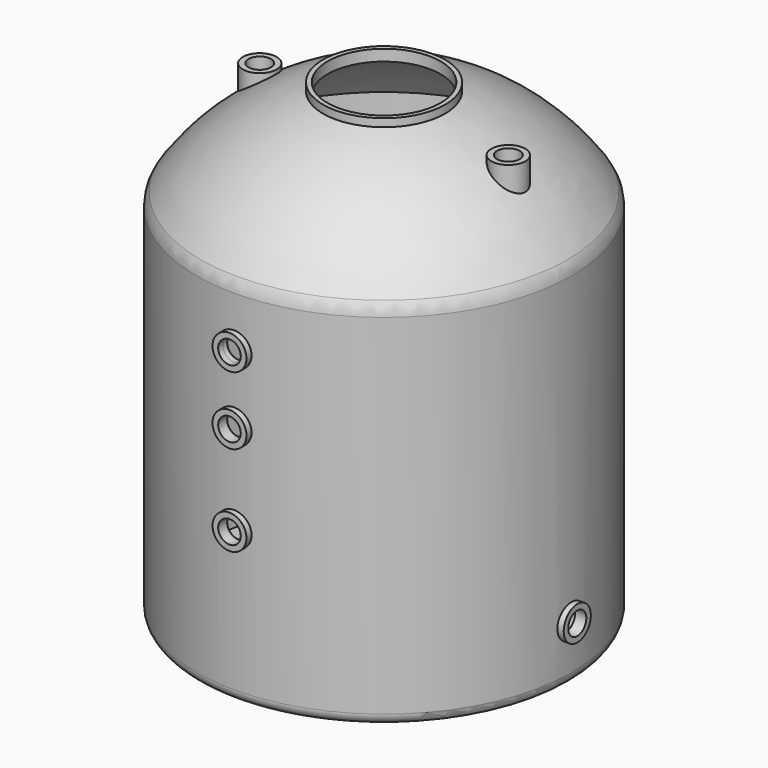
from build123d import *

# Parameters (mm, degrees)
F3_T      = 2
F9_DEPTH  = 12.5
F12_R     = 5
F13_DEPTH = 12.5
F14_R     = 7.5
F14_R_2   = 5
F15_DEPTH = 2.5
F19_R     = 10
F20_R     = 5
F24_R     = 5
F25_DEPTH = 40
F28_R     = 7.5
F28_R_2   = 5
F29_DEPTH = 10
F18_R     = 5
F30_DEPTH = 2.1554683744
F31_R     = 7.5
F31_R_2   = 5
F32_DEPTH = 2.5
F33_R     = 5
F34_DEPTH = 2.1554683744
F35_R     = 7.5
F35_R_2   = 5
F36_DEPTH = 2.5
F38_R     = 5
F39_DEPTH = 2.1554683744
F40_R     = 7.5
F40_R_2   = 5
F41_DEPTH = 2.5
F42_W     = 2.5
F42_H     = 1.25
F43_DEPTH = 3


with BuildPart() as f1:
    # F0 (on Front) → F1 (revolve)
    with BuildSketch(Plane.XZ):
        with BuildLine():
            Line((25, 99.9657286556), (0, 99.9657286556))
            Line((0, 99.9657286556), (0, -106.0342713444))
            Line((0, -106.0342713444), (81, -106.0342713444))
            Line((81, -106.0342713444), (81, 53.9657286556))
            ThreePointArc((81, 53.9657286556), (56.6710521362, 79.4798486465), (25, 94.9657286556))
            Line((25, 94.9657286556), (25, 99.9657286556))
        make_face()
    revolve(axis=Axis((0, 0, -3.0342713444), (0, 0, -1)))

    # F3
    f3_openings = [f1.faces().sort_by_distance(p)[0] for p in [
        (0, 0, 99.965729),
    ]]
    offset(amount=F3_T, openings=f3_openings, kind=Kind.INTERSECTION)

    # F8 (on offset) → F9 (cut, symmetric)
    with BuildSketch(Plane.XY.offset(61.5641335174)):
        with BuildLine():
            ThreePointArc((-43.2126436782, -4.9917358047), (-39.8642895048, -3.4324348785), (-38.5, 0))
            ThreePointArc((-38.5, 0), (-39.8642895048, 3.4324348785), (-43.2126436782, 4.9917358047))
            ThreePointArc((-43.2126436782, 4.9917358047), (-43.5, 0), (-43.2126436782, -4.9917358047))
        make_face()
        with BuildLine():
            ThreePointArc((-43.2126436782, 4.9917358047), (-39.8642895048, 3.4324348785), (-38.5, 0))
            ThreePointArc((-38.5, 0), (-39.8642895048, -3.4324348785), (-43.2126436782, -4.9917358047))
            ThreePointArc((-43.2126436782, -4.9917358047), (0, -43.5), (43.2126436782, -4.9917358047))
            ThreePointArc((43.2126436782, -4.9917358047), (38.5, 0), (43.2126436782, 4.9917358047))
            ThreePointArc((43.2126436782, 4.9917358047), (0, 43.5), (-43.2126436782, 4.9917358047))
        make_face()
        with BuildLine():
            ThreePointArc((-43.2126436782, -4.9917358047), (-43.5, 0), (-43.2126436782, 4.9917358047))
            ThreePointArc((-43.2126436782, 4.9917358047), (-48.5, 0), (-43.2126436782, -4.9917358047))
        make_face()
        with BuildLine():
            ThreePointArc((43.5, 0), (43.4281015012, 2.5), (43.2126436782, 4.9917358047))
            ThreePointArc((43.2126436782, 4.9917358047), (38.5, 0), (43.2126436782, -4.9917358047))
            ThreePointArc((43.2126436782, -4.9917358047), (43.4281015012, -2.5), (43.5, 0))
        make_face()
        with BuildLine():
            ThreePointArc((48.5, 0), (46.9324348785, 3.6357104952), (43.2126436782, 4.9917358047))
            ThreePointArc((43.2126436782, 4.9917358047), (43.4281015012, 2.5), (43.5, 0))
            ThreePointArc((43.5, 0), (43.4281015012, -2.5), (43.2126436782, -4.9917358047))
            ThreePointArc((43.2126436782, -4.9917358047), (46.9324348785, -3.6357104952), (48.5, 0))
        make_face()
    extrude(amount=F9_DEPTH, both=True, mode=Mode.SUBTRACT)

    # F12 (on plane+point) → F13 (cut, symmetric)
    with BuildSketch(Plane.XZ.offset(83)):
        with Locations((0, -40.4358664826)):
            Circle(F12_R)
        with Locations((0, -0.4358664826)):
            Circle(F12_R)
        with Locations((0, 29.5641335174)):
            Circle(F12_R)
    extrude(amount=F13_DEPTH, both=True, mode=Mode.SUBTRACT)

    # F14 (on plane+point) → F15 (join, symmetric)
    with BuildSketch(Plane.XZ.offset(83)):
        with Locations((0, -40.4358664826)):
            Circle(F14_R)
        with Locations((0, -40.4358664826)):
            Circle(F14_R_2, mode=Mode.SUBTRACT)
        with Locations((0, -0.4358664826)):
            Circle(F14_R)
        with Locations((0, -0.4358664826)):
            Circle(F14_R_2, mode=Mode.SUBTRACT)
        with Locations((0, 29.5641335174)):
            Circle(F14_R)
        with Locations((0, 29.5641335174)):
            Circle(F14_R_2, mode=Mode.SUBTRACT)
    extrude(amount=F15_DEPTH, both=True)

    # F19
    f19_edges = [f1.edges().sort_by_distance(p)[0] for p in [
        (-83, -0.000744, 54.567379),
    ]]
    fillet(f19_edges, radius=F19_R)

    # F20
    f20_edges = [f1.edges().sort_by_distance(p)[0] for p in [
        (-83, 0, -108.034271),
    ]]
    fillet(f20_edges, radius=F20_R)

    # F24 (on plane+point) → F25 (cut)
    with BuildSketch(Plane(origin=(0, 0, 54.5641335174), x_dir=(1, 0, 0), z_dir=(0, 0, -1))):
        with Locations((-55, 0)):
            Circle(F24_R)
        with Locations((55, 0)):
            Circle(F24_R)
    extrude(amount=-F25_DEPTH, mode=Mode.SUBTRACT)

    # F28 (on plane+point) → F29 (join, symmetric)
    with BuildSketch(Plane.XY.offset(79.4774252951)):
        with Locations((-55, 0)):
            Circle(F28_R)
        with Locations((-55, 0)):
            Circle(F28_R_2, mode=Mode.SUBTRACT)
        with Locations((55, 0)):
            Circle(F28_R)
        with Locations((55, 0)):
            Circle(F28_R_2, mode=Mode.SUBTRACT)
    extrude(amount=F29_DEPTH, both=True)

    # F18 (on plane+point) → F30 (cut, through all)
    with BuildSketch(Plane.YZ.offset(-83)):
        with Locations((0, -83.0342713444)):
            Circle(F18_R)
    extrude(amount=F30_DEPTH, mode=Mode.SUBTRACT)

    # F31 (on plane+point) → F32 (join, symmetric)
    with BuildSketch(Plane.YZ.offset(-83)):
        with Locations((0, -83.0342713444)):
            Circle(F31_R)
        with Locations((0, -83.0342713444)):
            Circle(F31_R_2, mode=Mode.SUBTRACT)
    extrude(amount=F32_DEPTH, both=True)

    # F33 (on line) → F34 (cut, through all)
    with BuildSketch(Plane.YZ.offset(83)):
        with Locations((0, -83.0342713444)):
            Circle(F33_R)
    extrude(amount=-F34_DEPTH, mode=Mode.SUBTRACT)

    # F35 (on line) → F36 (join, symmetric)
    with BuildSketch(Plane.YZ.offset(83)):
        with Locations((0, -83.0342713444)):
            Circle(F35_R)
        with Locations((0, -83.0342713444)):
            Circle(F35_R_2, mode=Mode.SUBTRACT)
    extrude(amount=F36_DEPTH, both=True)

    # F38 (on 3pt) → F39 (cut, through all)
    with BuildSketch(Plane(origin=(0, 83, 0), x_dir=(-1, 0, 0), z_dir=(0, 1, 0))):
        with Locations((0, -83.0342713444)):
            Circle(F38_R)
    extrude(amount=-F39_DEPTH, mode=Mode.SUBTRACT)

    # F40 (on 3pt) → F41 (join, symmetric)
    with BuildSketch(Plane(origin=(0, 83, 0), x_dir=(-1, 0, 0), z_dir=(0, 1, 0))):
        with Locations((0, -83.0342713444)):
            Circle(F40_R)
        with Locations((0, -83.0342713444)):
            Circle(F40_R_2, mode=Mode.SUBTRACT)
    extrude(amount=F41_DEPTH, both=True)

    # F42 (on face) → F43 (join)
    with BuildSketch(Plane(origin=(0, 0, -108.0342713444), x_dir=(1, 0, 0), z_dir=(0, 0, -1))):
        with Locations((51.6187950266, 49.7437950266)):
            Rectangle(F42_W, F42_H)
        with Locations((51.6187950266, 48.4937950266)):
            Rectangle(F42_W, F42_H)
    extrude(amount=-F43_DEPTH)


solid = f1.part
